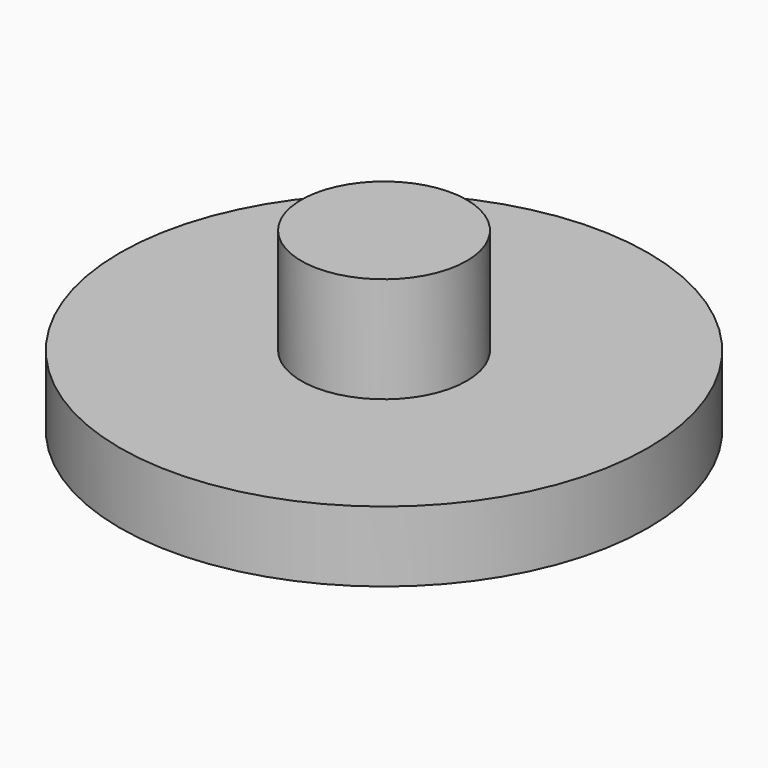
from build123d import *

# Parameters (mm, degrees)
F0_R     = 7.5
F1_DEPTH = 2
F2_R     = 2.35
F3_DEPTH = 3


# Not quite as in the source:
# - a feature names something its author has since deleted; it is built from what else it names


with BuildPart() as f1:
    # F0 (on Top) → F1 (new body)
    with BuildSketch(Plane.XY):
        with Locations((-37.0739325881, 46.6909147799)):
            Circle(F0_R)
    extrude(amount=F1_DEPTH)

    # F2 (on face) → F3 (join)
    with BuildSketch(Plane.XY.offset(2)):
        with Locations((-37.0739325881, 46.6909147799)):
            Circle(F2_R)
    extrude(amount=F3_DEPTH)


solid = f1.part
